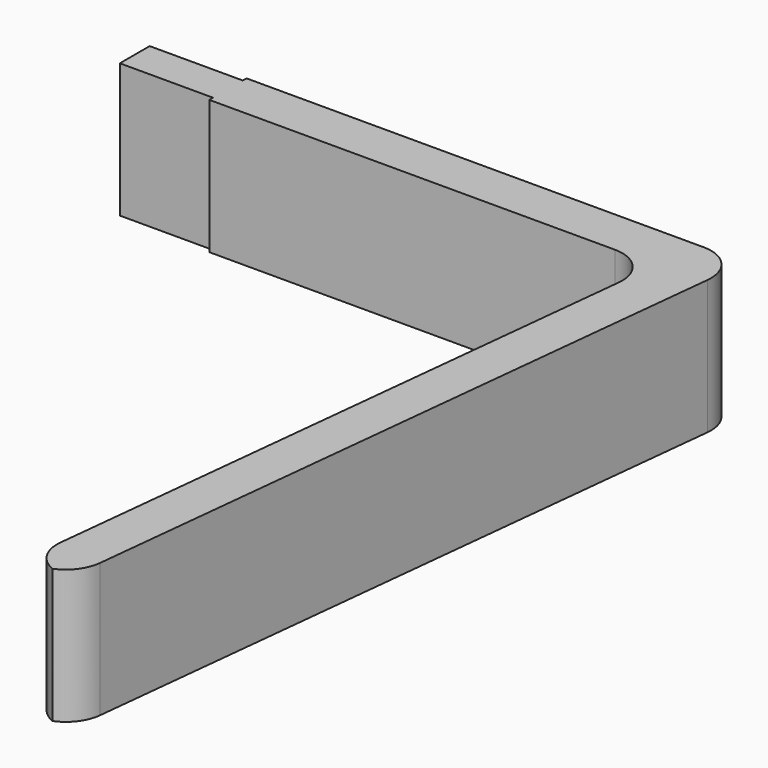
from build123d import *

# Parameters (mm, degrees)
F1_DEPTH    = 4.572
F2_T1_DEPTH = 4.572
F2_T3_DEPTH = 11.6353556042
F2_T5_DEPTH = 10.2806889376


# Not quite as in the source:
# - a fillet or chamfer that OpenCascade refuses, or shapes differently, is made with other operations: its cross-section is extruded or revolved along the edge and cut away or added


with BuildPart() as f1:
    # F0 (on Top) → F1 (new body)
    with BuildSketch(Plane.XY):
        Polygon((-16.9968333333, -0.15875), (-20.1718333333, -0.15875), (-20.1718333333, -1.42875), (-16.9968333333, -1.42875), (-16.9968333333, -1.5875), (-1.7568333333, -1.5875), (-4.2968333333, -25.4), (-2.7093333333, -25.4), (0, 0), (-16.9968333333, 0), align=None)
    extrude(amount=F1_DEPTH)

    # F2: fillet of radius 1.27 on 4 edges, made by hand

    # F2_s2 → F2_t1 (join)
    with BuildSketch(Plane.XY):
        with BuildLine():
            ThreePointArc((-1.9066682695, -2.9922025264), (-2.2250542944, -2.0084335151), (-3.1695044542, -1.5875))
            Line((-3.1695044542, -1.5875), (-1.7568333333, -1.5875))
            Line((-1.7568333333, -1.5875), (-1.9066682695, -2.9922025264))
        make_face()
    extrude(amount=F2_T1_DEPTH)

    # F2_s4 → F2_t3 (cut)
    with BuildSketch(Plane.XY.offset(-3.5316778021)):
        with BuildLine():
            ThreePointArc((-4.1469983972, -23.9952974736), (-3.8286123722, -24.9790664849), (-2.8841622125, -25.4))
            Line((-2.8841622125, -25.4), (-4.2968333333, -25.4))
            Line((-4.2968333333, -25.4), (-4.1469983972, -23.9952974736))
        make_face()
        with BuildLine():
            ThreePointArc((-0.1498349361, -1.4047025264), (-0.4682209611, -0.4209335151), (-1.4126711208, 0))
            Line((-1.4126711208, 0), (0, 0))
            Line((0, 0), (-0.1498349361, -1.4047025264))
        make_face()
    extrude(amount=F2_T3_DEPTH, mode=Mode.SUBTRACT)

    # F2_s6 → F2_t5 (cut)
    with BuildSketch(Plane.XY.offset(-2.8543444688)):
        with BuildLine():
            ThreePointArc((-3.8510711208, -25.4), (-3.002004636, -25.0744501597), (-2.5882349361, -24.2647025264))
            Line((-2.5882349361, -24.2647025264), (-2.7093333333, -25.4))
            Line((-2.7093333333, -25.4), (-3.8510711208, -25.4))
        make_face()
    extrude(amount=F2_T5_DEPTH, mode=Mode.SUBTRACT)


solid = f1.part
